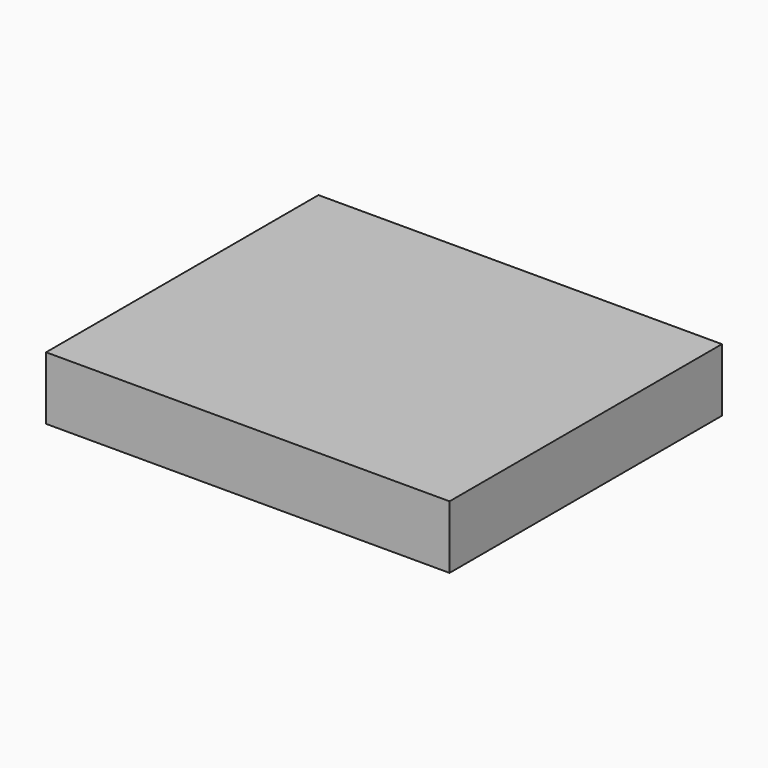
from build123d import *

# Parameters (mm, degrees)
F0_W     = 320
F0_H     = 50
F1_DEPTH = 270
F2_T     = -5
F3_W     = 70
F3_H     = 20
F4_DEPTH = 25
F5_F1_R  = 2
F5_F2_R  = 2


with BuildPart() as f1:
    # F0 (on Front) → F1 (new body)
    with BuildSketch(Plane.XZ):
        with Locations((-36.4068159834, 46.1331414707)):
            Rectangle(F0_W, F0_H)
    extrude(amount=F1_DEPTH)

    # F2
    f2_openings = [f1.faces().sort_by_distance(p)[0] for p in [
        (-36.406816, -135, 21.133141),
    ]]
    offset(amount=F2_T, openings=f2_openings)

    # F3 (on face) → F4 (cut)
    with BuildSketch(Plane(origin=(0, 0, 0), x_dir=(-1, 0, 0), z_dir=(0, 1, 0))):
        with Locations((-48.5931840166, 31.1331414707)):
            Rectangle(F3_W, F3_H)
    extrude(amount=-F4_DEPTH, mode=Mode.SUBTRACT)

    # F5: fillet of radius 2 on 6 edges, made by hand

    # F5_f1
    f5_f1_edges = [f1.edges().sort_by_distance(p)[0] for p in [
        (83.5931840166, -2.5, 41.1331414707),
        (13.5931840166, -2.5, 41.1331414707),
    ]]
    fillet(f5_f1_edges, radius=F5_F1_R)

    # F5_f2
    f5_f2_edges = [f1.edges().sort_by_distance(p)[0] for p in [
        (83.5931840166, -2.5, 21.1331414707),
        (13.5931840166, -2.5, 21.1331414707),
        (48.5931840166, 0, 41.1331414707),
        (48.5931840166, -5, 41.1331414707),
        (83.007397579, -5, 40.5473550331),
        (14.1789704543, -5, 40.5473550331),
        (14.1789704543, 0, 40.5473550331),
        (83.007397579, 0, 40.5473550331),
    ]]
    fillet(f5_f2_edges, radius=F5_F2_R)


solid = f1.part
